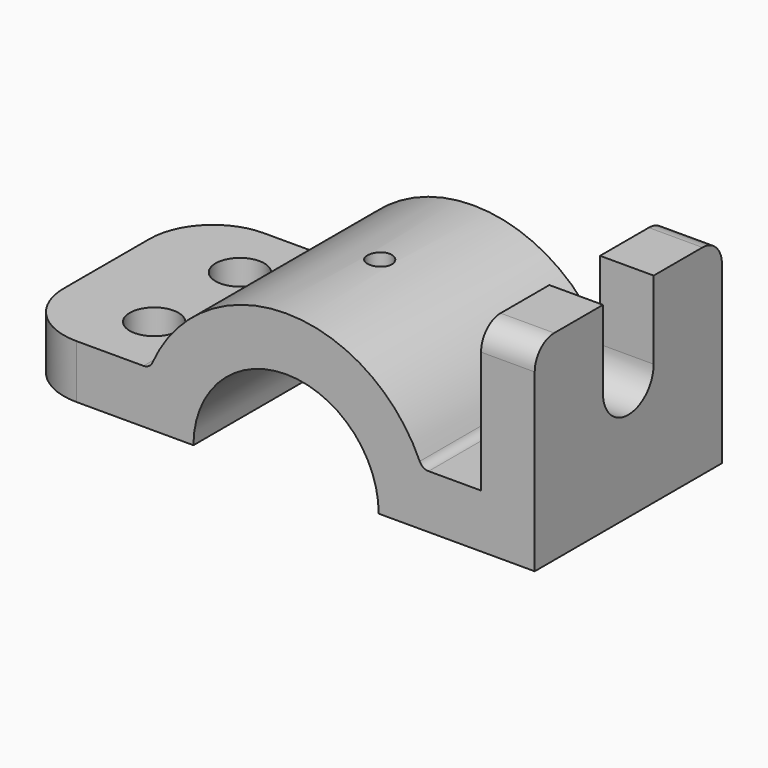
from build123d import *

# Parameters (mm, degrees)
F0_W     = 11
F0_H     = 30
F1_DEPTH = 24
F3_DEPTH = 17.3
F5_D     = 10
F6_D     = 5
F7_R     = 13
F8_R     = 5
F9_R     = 2


with BuildPart() as f1:
    # F0 (on Front) → F1 (new body, symmetric)
    with BuildSketch(Plane.XZ):
        with BuildLine():
            Line((-56, 0), (-30, 0))
            ThreePointArc((-30, 0), (-29.4730143031, 5.5983415304), (-27.9105714739, 11))
            Line((-27.9105714739, 11), (-56, 11))
            Line((-56, 11), (-56, 0))
        make_face()
        with BuildLine():
            Line((-30, 0), (-19, 0))
            ThreePointArc((-19, 0), (-18.1017503893, 5.7729223833), (-15.4919333848, 11))
            Line((-15.4919333848, 11), (-27.9105714739, 11))
            ThreePointArc((-27.9105714739, 11), (-29.4730143031, 5.5983415304), (-30, 0))
        make_face()
        with BuildLine():
            ThreePointArc((-15.4919333848, 11), (0, 19), (15.4919333848, 11))
            Line((15.4919333848, 11), (27.9105714739, 11))
            ThreePointArc((27.9105714739, 11), (0, 30), (-27.9105714739, 11))
            Line((-27.9105714739, 11), (-15.4919333848, 11))
        make_face()
        with BuildLine():
            ThreePointArc((15.4919333848, 11), (18.1017503893, 5.7729223833), (19, 0))
            Line((19, 0), (30, 0))
            ThreePointArc((30, 0), (29.4730143031, 5.5983415304), (27.9105714739, 11))
            Line((27.9105714739, 11), (15.4919333848, 11))
        make_face()
        with BuildLine():
            ThreePointArc((27.9105714739, 11), (29.4730143031, 5.5983415304), (30, 0))
            Line((30, 0), (51, 0))
            Line((51, 0), (51, 11))
            Line((51, 11), (40, 11))
            Line((40, 11), (27.9105714739, 11))
        make_face()
        with Locations((45.5, 26)):
            Rectangle(F0_W, F0_H)
    extrude(amount=F1_DEPTH, both=True)

    # F2 (on face) → F3 (cut)
    with BuildSketch(Plane.YZ.offset(51)):
        with BuildLine():
            ThreePointArc((-6.5, 25), (0, 18.5), (6.5, 25))
            ThreePointArc((6.5, 25), (0, 31.5), (-6.5, 25))
        make_face()
        with BuildLine():
            ThreePointArc((-6.5, 25), (0, 31.5), (6.5, 25))
            Line((6.5, 25), (6.5, 41))
            Line((6.5, 41), (-6.5, 41))
            Line((-6.5, 41), (-6.5, 25))
        make_face()
    extrude(amount=-F3_DEPTH, mode=Mode.SUBTRACT)

    # F5 (through all)
    with Locations(Plane(origin=(0, 0, 0), x_dir=(1, 0, 0), z_dir=(0, 0, -1))):
        with Locations((-37.4579249547, -11), (-37.4579249547, 11)):
            Hole(F5_D / 2)

    # F6 (through all)
    with Locations(Plane(origin=(0, 0, 0), x_dir=(1, 0, 0), z_dir=(0, 0, -1))):
        with Locations((0, 0)):
            Hole(F6_D / 2)

    # F7
    f7_edges = [f1.edges().sort_by_distance(p)[0] for p in [
        (-56, -24, 5.5),
        (-56, 24, 5.5),
    ]]
    fillet(f7_edges, radius=F7_R)

    # F8
    f8_edges = [f1.edges().sort_by_distance(p)[0] for p in [
        (45.5, 24, 41),
        (45.5, -24, 41),
    ]]
    fillet(f8_edges, radius=F8_R)

    # F9
    f9_edges = [f1.edges().sort_by_distance(p)[0] for p in [
        (27.910571, 0, 11),
        (-27.910571, 0, 11),
    ]]
    fillet(f9_edges, radius=F9_R)


solid = f1.part
